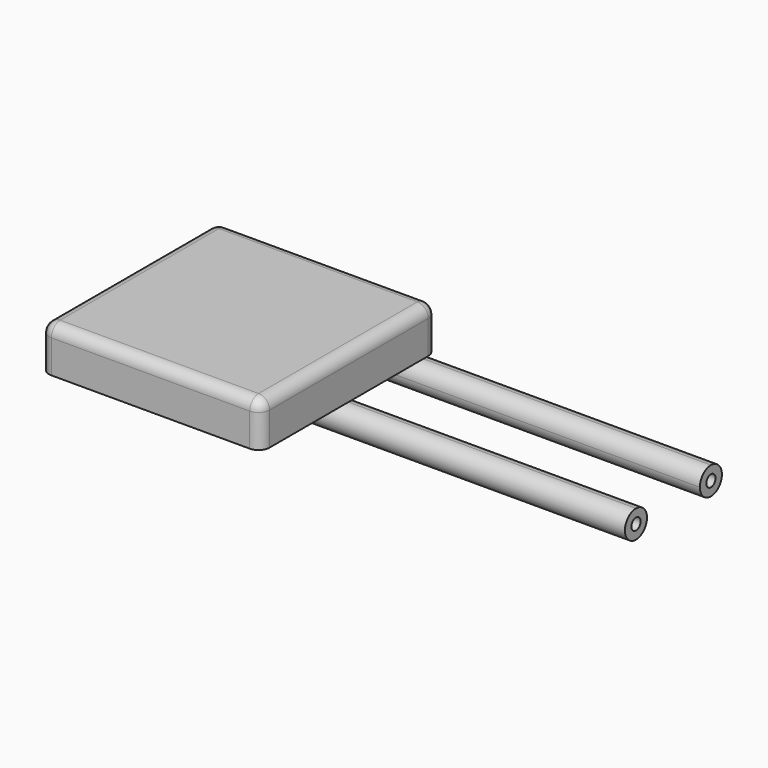
from build123d import *

# Parameters (mm, degrees)
F1_DEPTH = 400
F0_R     = 10.5
F2_DEPTH = 922
F3_R     = 20


# Not quite as in the source:
# - a feature names something its author has since deleted; it is built from what else it names


with BuildPart() as f1:
    # F0 (on Right) → F1 (new body)
    with BuildSketch(Plane.YZ):
        Polygon((-258.8667411456, -8.3345091114), (-60.1131648569, -8.3345091114), (109.8868350748, -8.3345091114), (141.1332431091, -8.3345091114), (141.1332431091, 71.6654908886), (-258.8667411456, 71.6654908886), align=None)
    extrude(amount=F1_DEPTH)

    # F3
    f3_edges = [f1.edges().sort_by_distance(p)[0] for p in [
        (200, -258.866741, 71.665491),
        (400, -58.866749, 71.665491),
        (200, 141.133243, 71.665491),
        (0, -58.866749, 71.665491),
        (400, 141.133243, 31.665491),
        (0, 141.133243, 31.665491),
        (400, -258.866741, 31.665491),
        (0, -258.866741, 31.665491),
    ]]
    fillet(f3_edges, radius=F3_R)


with BuildPart() as f2:
    # F0 (on Right) → F2 (new body)
    with BuildSketch(Plane.YZ):
        with BuildLine():
            ThreePointArc((-60.1131648569, -8.3345091114), (-77.790834479, -51.0121786169), (-35.1131649252, -33.3345091114))
            ThreePointArc((-35.1131649252, -33.3345091114), (-42.4354953714, -15.6568396059), (-60.1131648569, -8.3345091114))
        make_face()
        with Locations((-60.1131649252, -33.3345091114)):
            Circle(F0_R, mode=Mode.SUBTRACT)
    extrude(amount=F2_DEPTH)


with BuildPart() as f2b:
    # F0 (on Right) → F2, piece 2 (new body)
    with BuildSketch(Plane.YZ):
        with BuildLine():
            ThreePointArc((109.8868350748, -8.3345091114), (92.2091655451, -15.6568395818), (84.8868350748, -33.3345091114))
            Line((84.8868350748, -33.3345091114), (99.3868350748, -33.3345091114))
            ThreePointArc((99.3868350748, -33.3345091114), (109.8868350748, -22.8345091114), (120.3868350748, -33.3345091114))
            Line((120.3868350748, -33.3345091114), (134.8868350748, -33.3345091114))
            ThreePointArc((134.8868350748, -33.3345091114), (127.5645046045, -15.6568395818), (109.8868350748, -8.3345091114))
        make_face()
        with BuildLine():
            Line((99.3868350748, -33.3345091114), (84.8868350748, -33.3345091114))
            ThreePointArc((84.8868350748, -33.3345091114), (109.8868350748, -58.3345091114), (134.8868350748, -33.3345091114))
            Line((134.8868350748, -33.3345091114), (120.3868350748, -33.3345091114))
            ThreePointArc((120.3868350748, -33.3345091114), (109.8868350748, -43.8345091114), (99.3868350748, -33.3345091114))
        make_face()
    extrude(amount=F2_DEPTH)


solid = Compound([f1.part, f2.part, f2b.part])
